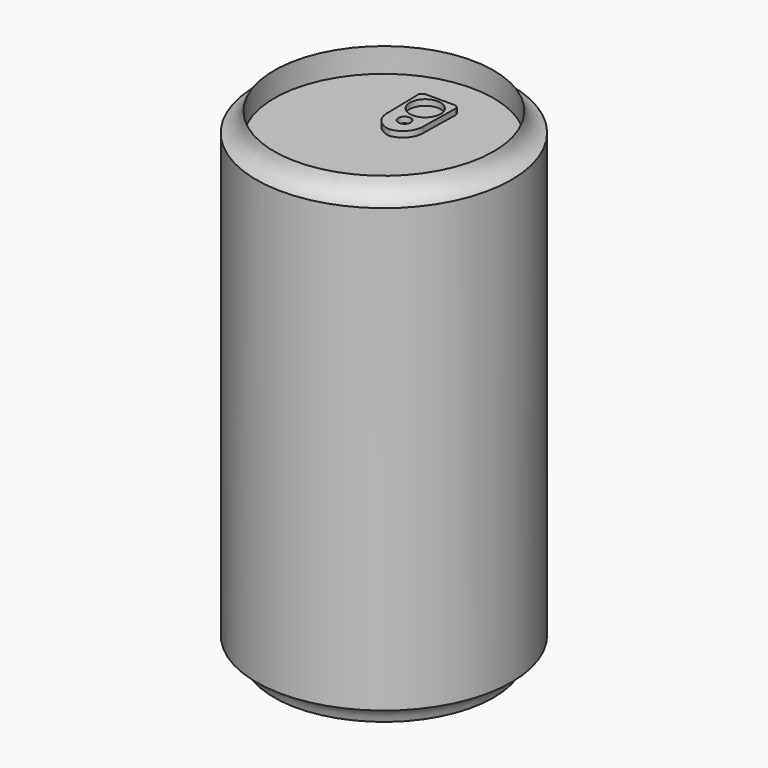
from build123d import *

# Parameters (mm, degrees)
F0_R      = 33.15
F1_DEPTH  = 57.5
F3_DEPTH  = 5
F8_DEPTH  = 5
F9_DEPTH  = 3.048
F10_R     = 28.5244197483
F11_DEPTH = 6.35
F14_DEPTH = 1.5


# Not quite as in the source:
# - a feature names something its author has since deleted; it is built from what else it names


with BuildPart() as f1:
    # F0 (on Top) → F1 (new body, symmetric)
    with BuildSketch(Plane.XY):
        Circle(F0_R)
    extrude(amount=F1_DEPTH, both=True)

    # F2 (on face) → F3 (join)
    with BuildSketch(Plane.XY.offset(57.5)):
        with BuildLine():
            ThreePointArc((27.5449306971, 7.4107567004), (-28.2784872926, -3.7376032987), (28.5244197483, 0))
            ThreePointArc((28.5244197483, 0), (28.2784872926, 3.7376032987), (27.5449306971, 7.4107567004))
        make_face()
        with BuildLine():
            Line((-3.6688328255, 16.6036896408), (0, 16.6036896408))
            Line((0, 16.6036896408), (3.6688328255, 16.6036896408))
            ThreePointArc((3.6688328255, 16.6036896408), (4.3933325809, 16.3940702991), (4.8939753324, 15.8299807676))
            Line((4.8939753324, 15.8299807676), (4.6938681044, 5.1092766225))
            ThreePointArc((4.6938681044, 5.1092766225), (3.3149072999, 1.6653658978), (0, 0))
            ThreePointArc((0, 0), (-3.3149072999, 1.6653658978), (-4.6938681044, 5.1092766225))
            Line((-4.6938681044, 5.1092766225), (-4.8939753324, 15.8299807676))
            ThreePointArc((-4.8939753324, 15.8299807676), (-4.3933325809, 16.3940702991), (-3.6688328255, 16.6036896408))
        make_face(mode=Mode.SUBTRACT)
    extrude(amount=F3_DEPTH)

    # F7: F6 across plane


with BuildPart() as f6:
    # F4 (on Front) → F6 (revolve)
    with BuildSketch(Plane.XZ):
        with BuildLine():
            add(Edge.make_bspline(
                [(28.5244197483, 62.5), (28.9434660226, 59.606384486), (31.2671773136, 57.7946938574), (33.15, 57.5)],
                knots=[0, 0, 0, 0, 6.8114603915, 6.8114603915, 6.8114603915, 6.8114603915], degree=3))
            Line((28.5244197483, 62.5), (28.5244197483, 57.5))
            Line((28.5244197483, 57.5), (33.15, 57.5))
        make_face()
    revolve(axis=Axis((0, 0, 67.1579949558), (0, 0, 1)))


with BuildPart() as f1_1:
    add(f1.part)
    add(f6.part.mirror(Plane.XY))

    # F8 (add): a face of the model
    f8_faces = [f1_1.faces().sort_by_distance(p)[0] for p in [
        (0, 0, -57.5),
    ]]
    extrude(f8_faces, amount=F8_DEPTH)

    # F9 (add): a face of the model
    f9_faces = [f1_1.faces().sort_by_distance(p)[0] for p in [
        (0, -0.5407612008, 62.5),
    ]]

    add(f6.part)  # F9 merges F6
    extrude(f9_faces, amount=-F9_DEPTH)

    # F10 (on face) → F11 (cut)
    with BuildSketch(Plane.XY.offset(62.5)):
        Circle(F10_R)
    extrude(amount=-F11_DEPTH, mode=Mode.SUBTRACT)

    # F13 (on face) → F14 (join)
    with BuildSketch(Plane.XY.offset(56.15)):
        with BuildLine():
            Line((3.6663445585, 18.275173819), (-0.002488267, 18.275173819))
            Line((-0.002488267, 18.275173819), (-3.6713210925, 18.275173819))
            ThreePointArc((-3.6713210925, 18.275173819), (-4.395820848, 18.0655544773), (-4.8964635994, 17.5014649459))
            Line((-4.8964635994, 17.5014649459), (-4.6963563714, 6.7807608008))
            ThreePointArc((-4.6963563714, 6.7807608008), (-3.3173955669, 3.336850076), (-0.002488267, 1.6714841783))
            ThreePointArc((-0.002488267, 1.6714841783), (3.3124190329, 3.336850076), (4.6913798374, 6.7807608008))
            Line((4.6913798374, 6.7807608008), (4.8914870654, 17.5014649459))
            ThreePointArc((4.8914870654, 17.5014649459), (4.3908443139, 18.0655544773), (3.6663445585, 18.275173819))
        make_face()
        with BuildLine():
            ThreePointArc((-0.002488267, 8.3136439422), (1.6104378587, 6.7007178165), (-0.002488267, 5.0877916907))
            ThreePointArc((-0.002488267, 5.0877916907), (-1.6154143928, 6.7007178165), (-0.002488267, 8.3136439422))
        make_face(mode=Mode.SUBTRACT)
        with BuildLine():
            ThreePointArc((-0.002488267, 17.4195373118), (3.997511733, 13.4195373118), (-0.002488267, 9.4195373118))
            ThreePointArc((-0.002488267, 9.4195373118), (-4.002488267, 13.4195373118), (-0.002488267, 17.4195373118))
        make_face(mode=Mode.SUBTRACT)
    extrude(amount=F14_DEPTH)


solid = f1_1.part
